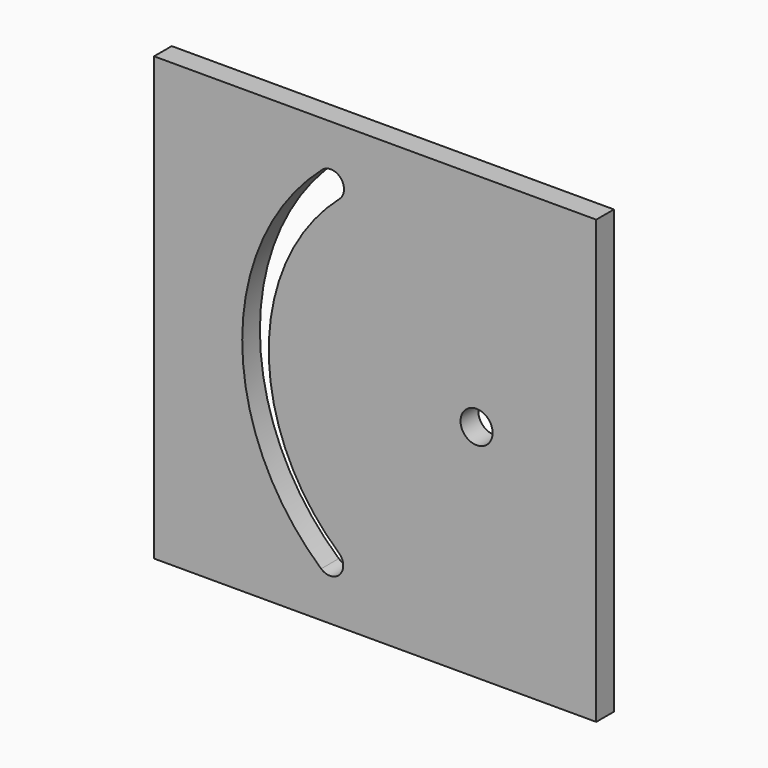
from build123d import *

# Parameters (mm, degrees)
F0_W     = 200
F0_H     = 200
F0_R     = 7.25
F1_DEPTH = 10


with BuildPart() as f1:
    # F0 (on Front) → F1 (new body)
    with BuildSketch(Plane.XZ):
        Rectangle(F0_W, F0_H)
        with BuildLine():
            ThreePointArc((-24.4348083961, -79.4901646735), (-60.1255414788, 0.098775478), (-24.0407608064, 79.5098353265))
            ThreePointArc((-24.0407608064, 79.5098353265), (-15.5734786606, 78.9574468193), (-16.1258671678, 70.4901646735))
            ThreePointArc((-16.1258671678, 70.4901646735), (-48.12557833, 0.0690361286), (-16.4753055963, -70.5098353265))
            ThreePointArc((-16.4753055963, -70.5098353265), (-15.9648923227, -78.9797513999), (-24.4348083961, -79.4901646735))
        make_face(mode=Mode.SUBTRACT)
        with Locations((45.8741330018, -0.1639221083)):
            Circle(F0_R, mode=Mode.SUBTRACT)
    extrude(amount=F1_DEPTH)


solid = f1.part
